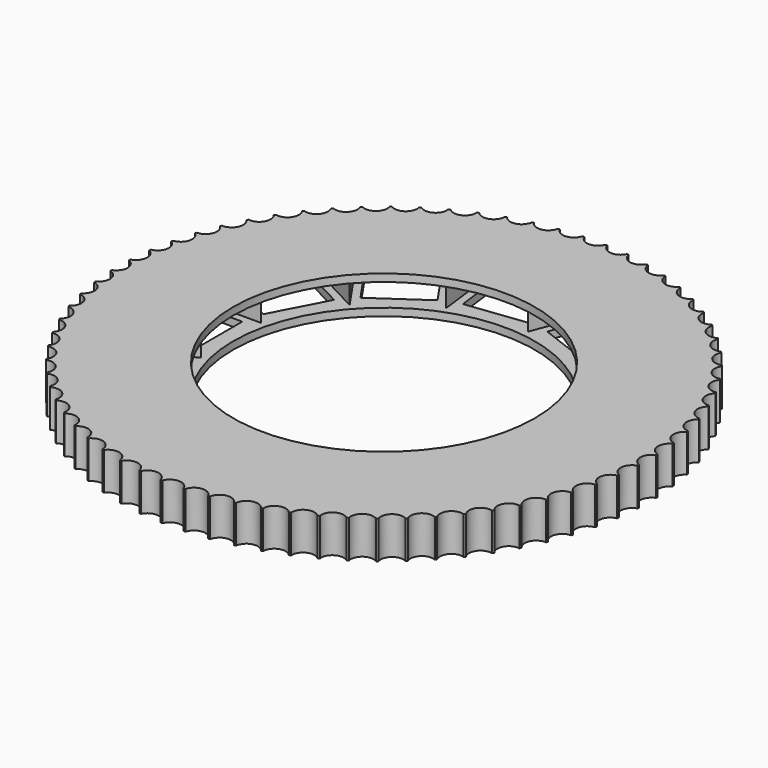
from build123d import *

# Parameters (mm, degrees)
F1_R          = 35
F1_R_2        = 20
F2_DEPTH      = 4
F2_DEPTH_BACK = 1
F0_W          = 10
F0_H          = 8
F3_DEPTH      = 3
F3_DEPTH_BACK = 1
F4_DEPTH      = 3
F5_R          = 1.5
F6_DEPTH      = 4.001
F6_DEPTH_BACK = 1.001


# Not quite as in the source:
# - a feature of the source that left no trace in its solid (it failed there, or was rolled back) is left out


with BuildPart() as f2:
    # F1 (on Top) → F2 (new body, two sides)
    with BuildSketch(Plane.XY) as f2_sk:
        Circle(F1_R)
        Circle(F1_R_2, mode=Mode.SUBTRACT)
    extrude(amount=F2_DEPTH)
    extrude(f2_sk.sketch, amount=-F2_DEPTH_BACK)

    # F0 (on Top) → F3 (cut, two sides)
    with BuildSketch(Plane.XY) as f3_sk:
        with Locations((-27, 0)):
            Rectangle(F0_W, F0_H)
        Polygon((-21.3389252525, -6.6820856824), (-30.1934855091, -11.3293174028), (-26.4757001327, -18.412965608), (-17.6211398762, -13.7657338876), align=None)
        Polygon((-15.7893598917, -15.8333860627), (-21.470007359, -24.0632247217), (-14.8861364318, -28.6077426955), (-9.2054889645, -20.3779040366), align=None)
        Polygon((-6.622642462, -21.3574485091), (-7.8280092646, -31.2845372501), (0.1136617282, -32.2488306922), (1.3190285308, -22.3217419512), align=None)
        Polygon((4.0612425442, -21.9887768872), (7.6072914146, -31.3389393141), (15.0874213561, -28.5021002178), (11.5413724857, -19.1519377909), align=None)
        Polygon((13.8147458268, -17.582741474), (21.2998533085, -24.2139680564), (26.6048345744, -18.225882071), (19.1197270927, -11.5946554886), align=None)
        Polygon((20.4034573262, -9.148711884), (30.1128755005, -11.5418685269), (32.0274008148, -3.7743339875), (22.3179826405, -1.3811773446), align=None)
        Polygon((22.3179826405, 1.3811773446), (32.0274008148, 3.7743339875), (30.1128755005, 11.5418685269), (20.4034573262, 9.148711884), align=None)
        Polygon((19.1197270927, 11.5946554886), (26.6048345744, 18.225882071), (21.2998533085, 24.2139680564), (13.8147458268, 17.582741474), align=None)
        Polygon((11.5413724857, 19.1519377909), (15.0874213561, 28.5021002178), (7.6072914146, 31.3389393141), (4.0612425442, 21.9887768872), align=None)
        Polygon((1.3190285308, 22.3217419512), (0.1136617282, 32.2488306922), (-7.8280092646, 31.2845372501), (-6.622642462, 21.3574485091), align=None)
        Polygon((-9.2054889645, 20.3779040366), (-14.8861364318, 28.6077426955), (-21.470007359, 24.0632247217), (-15.7893598917, 15.8333860627), align=None)
        Polygon((-17.6211398762, 13.7657338876), (-26.4757001327, 18.412965608), (-30.1934855091, 11.3293174028), (-21.3389252525, 6.6820856824), align=None)
    extrude(amount=F3_DEPTH, mode=Mode.SUBTRACT)
    extrude(f3_sk.sketch, amount=-F3_DEPTH_BACK, mode=Mode.SUBTRACT)

    # F0 (on Top) → F4 (cut)
    with BuildSketch(Plane.XY):
        Polygon((-20.2857974282, 5), (-33, 5), (-33, -5), (-20.2857974282, -5), (-10.7590933717, 0), align=None)
        with Locations((-27, 0)):
            Rectangle(F0_W, F0_H, mode=Mode.SUBTRACT)
        Polygon((-31.5436647068, 10.9085845492), (-20.2857974282, 5), (-9.5267040565, 5), (-15.6385657078, 13.8545602565), (-26.8964329863, 19.7631448057), align=None)
        Polygon((-30.1934855091, 11.3293174028), (-26.4757001327, 18.412965608), (-17.6211398762, 13.7657338876), (-21.3389252525, 6.6820856824), align=None, mode=Mode.SUBTRACT)
        Polygon((-9.5267040565, 5), (-20.2857974282, 5), (-10.7590933717, 0), (-7.3209820639, 1.8044600144), align=None)
        Polygon((-15.6385657078, 13.8545602565), (-9.5267040565, 5), (-5.6438333004, 5), (-6.1118616512, 8.8545602565), align=None)
        Polygon((-7.3209820639, -1.8044600144), (-10.7590933717, 0), (-20.2857974282, -5), (-9.5267040565, -5), align=None)
        Polygon((-9.5267040565, -5), (-20.2857974282, -5), (-31.5436647068, -10.9085845492), (-26.8964329863, -19.7631448057), (-15.6385657078, -13.8545602565), align=None)
        Polygon((-26.4757001327, -18.412965608), (-30.1934855091, -11.3293174028), (-21.3389252525, -6.6820856824), (-17.6211398762, -13.7657338876), align=None, mode=Mode.SUBTRACT)
        Polygon((-22.8610559716, 24.3181438408), (-15.6385657078, 13.8545602565), (-6.1118616512, 8.8545602565), (-7.4087270488, 19.5352077238), (-14.6312173127, 29.9987913081), align=None)
        Polygon((-21.470007359, 24.0632247217), (-14.8861364318, 28.6077426955), (-9.2054889645, 20.3779040366), (-15.7893598917, 15.8333860627), align=None, mode=Mode.SUBTRACT)
        Polygon((-5.6438333004, -5), (-9.5267040565, -5), (-15.6385657078, -13.8545602565), (-6.1118616512, -8.8545602565), align=None)
        Polygon((-7.4087270488, 19.5352077238), (-6.1118616512, 8.8545602565), (-2.6737503434, 7.0501002421), (-1.2968653976, 10.6806474673), align=None)
        Polygon((-6.1118616512, -8.8545602565), (-15.6385657078, -13.8545602565), (-22.8610559716, -24.3181438408), (-14.6312173127, -29.9987913081), (-7.4087270488, -19.5352077238), align=None)
        Polygon((-14.8861364318, -28.6077426955), (-21.470007359, -24.0632247217), (-15.7893598917, -15.8333860627), (-9.2054889645, -20.3779040366), align=None, mode=Mode.SUBTRACT)
        Polygon((-8.9412548189, 32.156709444), (-7.4087270488, 19.5352077238), (-1.2968653976, 10.6806474673), (2.5183616922, 20.7405745264), (0.9858339221, 33.3620762465), align=None)
        Polygon((-7.8280092646, 31.2845372501), (0.1136617282, 32.2488306922), (1.3190285308, 22.3217419512), (-6.622642462, 21.3574485091), align=None, mode=Mode.SUBTRACT)
        Polygon((-2.6737503434, -7.0501002421), (-6.1118616512, -8.8545602565), (-7.4087270488, -19.5352077238), (-1.2968653976, -10.6806474673), align=None)
        Polygon((2.5183616922, 20.7405745264), (-1.2968653976, 10.6806474673), (0.9088565951, 7.4851074817), (3.8152270897, 10.0599270591), align=None)
        Polygon((-1.2968653976, -10.6806474673), (-7.4087270488, -19.5352077238), (-8.9412548189, -32.156709444), (0.9858339221, -33.3620762465), (2.5183616922, -20.7405745264), align=None)
        Polygon((0.1136617282, -32.2488306922), (-7.8280092646, -31.2845372501), (-6.622642462, -21.3574485091), (1.3190285308, -22.3217419512), align=None, mode=Mode.SUBTRACT)
        Polygon((7.026880059, 32.6285604438), (2.5183616922, 20.7405745264), (3.8152270897, 10.0599270591), (11.868524119, 17.194525656), (16.3770424858, 29.0825115734), align=None)
        Polygon((7.6072914146, 31.3389393141), (15.0874213561, 28.5021002178), (11.5413724857, 19.1519377909), (4.0612425442, 21.9887768872), align=None, mode=Mode.SUBTRACT)
        Polygon((0.9088565951, -7.4851074817), (-1.2968653976, -10.6806474673), (2.5183616922, -20.7405745264), (3.8152270897, -10.0599270591), align=None)
        Polygon((11.868524119, 17.194525656), (3.8152270897, 10.0599270591), (4.2832554405, 6.2053668026), (8.0532970293, 7.1345985969), align=None)
        Polygon((3.8152270897, -10.0599270591), (2.5183616922, -20.7405745264), (7.026880059, -32.6285604438), (16.3770424858, -29.0825115734), (11.868524119, -17.194525656), align=None)
        Polygon((15.0874213561, -28.5021002178), (7.6072914146, -31.3389393141), (4.0612425442, -21.9887768872), (11.5413724857, -19.1519377909), align=None, mode=Mode.SUBTRACT)
        Polygon((21.3852413984, 25.6256014628), (11.868524119, 17.194525656), (8.0532970293, 7.1345985969), (18.4997507014, 9.7094181743), (28.0164679809, 18.1404939811), align=None)
        Polygon((21.2998533085, 24.2139680564), (26.6048345744, 18.225882071), (19.1197270927, 11.5946554886), (13.8147458268, 17.582741474), align=None, mode=Mode.SUBTRACT)
        Polygon((4.2832554405, -6.2053668026), (3.8152270897, -10.0599270591), (11.868524119, -17.194525656), (8.0532970293, -7.1345985969), align=None)
        Polygon((18.4997507014, 9.7094181743), (8.0532970293, 7.1345985969), (6.6764120834, 3.5040513717), (10.4464536722, 2.5748195774), align=None)
        Polygon((8.0532970293, -7.1345985969), (11.868524119, -17.194525656), (21.3852413984, -25.6256014628), (28.0164679809, -18.1404939811), (18.4997507014, -9.7094181743), align=None)
        Polygon((26.6048345744, -18.225882071), (21.2998533085, -24.2139680564), (13.8147458268, -17.582741474), (19.1197270927, -11.5946554886), align=None, mode=Mode.SUBTRACT)
        Polygon((30.8445016536, 12.7521260086), (18.4997507014, 9.7094181743), (10.4464536722, 2.5748195774), (20.8929073443, 0), (33.2376582965, 3.0427078344), align=None)
        Polygon((30.1128755005, 11.5418685269), (32.0274008148, 3.7743339875), (22.3179826405, 1.3811773446), (20.4034573262, 9.148711884), align=None, mode=Mode.SUBTRACT)
        Polygon((6.6764120834, -3.5040513717), (8.0532970293, -7.1345985969), (18.4997507014, -9.7094181743), (10.4464536722, -2.5748195774), align=None)
        Polygon((20.8929073443, 0), (10.4464536722, 2.5748195774), (7.5400831775, 0), (10.4464536722, -2.5748195774), align=None)
        Polygon((10.4464536722, -2.5748195774), (18.4997507014, -9.7094181743), (30.8445016536, -12.7521260086), (33.2376582965, -3.0427078344), (20.8929073443, 0), align=None)
        Polygon((32.0274008148, -3.7743339875), (30.1128755005, -11.5418685269), (20.4034573262, -9.148711884), (22.3179826405, -1.3811773446), align=None, mode=Mode.SUBTRACT)
    extrude(amount=F4_DEPTH, mode=Mode.SUBTRACT)

    # F5 (on Top) → F6 (cut, two sides)
    with BuildSketch(Plane.XY) as f6_sk:
        with Locations((-35.5, 0)):
            Circle(F5_R)
        with Locations((-35.3649117823, -3.0940288675)):
            Circle(F5_R)
        with Locations((-34.9606752319, -6.1645103072)):
            Circle(F5_R)
        with Locations((-34.2903668333, -9.1880761011)):
            Circle(F5_R)
        with Locations((-33.3590880379, -12.1417150881)):
            Circle(F5_R)
        with Locations((-32.1739264398, -15.0029482918)):
            Circle(F5_R)
        with Locations((-30.7439018343, -17.75)):
            Circle(F5_R)
        with Locations((-29.0798975723, -20.3619634905)):
            Circle(F5_R)
        with Locations((-27.1945777307, -22.8189601439)):
            Circle(F5_R)
        with Locations((-25.1022907321, -25.1022907321)):
            Circle(F5_R)
        with Locations((-22.8189601439, -27.1945777307)):
            Circle(F5_R)
        with Locations((-20.3619634905, -29.0798975723)):
            Circle(F5_R)
        with Locations((-17.75, -30.7439018343)):
            Circle(F5_R)
        with Locations((-15.0029482918, -32.1739264398)):
            Circle(F5_R)
        with Locations((-12.1417150881, -33.3590880379)):
            Circle(F5_R)
        with Locations((-9.1880761011, -34.2903668333)):
            Circle(F5_R)
        with Locations((-6.1645103072, -34.9606752319)):
            Circle(F5_R)
        with Locations((-3.0940288675, -35.3649117823)):
            Circle(F5_R)
        with Locations((0, -35.5)):
            Circle(F5_R)
        with Locations((3.0940288675, -35.3649117823)):
            Circle(F5_R)
        with Locations((6.1645103072, -34.9606752319)):
            Circle(F5_R)
        with Locations((9.1880761011, -34.2903668333)):
            Circle(F5_R)
        with Locations((12.1417150881, -33.3590880379)):
            Circle(F5_R)
        with Locations((15.0029482918, -32.1739264398)):
            Circle(F5_R)
        with Locations((17.75, -30.7439018343)):
            Circle(F5_R)
        with Locations((20.3619634905, -29.0798975723)):
            Circle(F5_R)
        with Locations((22.8189601439, -27.1945777307)):
            Circle(F5_R)
        with Locations((25.1022907321, -25.1022907321)):
            Circle(F5_R)
        with Locations((27.1945777307, -22.8189601439)):
            Circle(F5_R)
        with Locations((29.0798975723, -20.3619634905)):
            Circle(F5_R)
        with Locations((30.7439018343, -17.75)):
            Circle(F5_R)
        with Locations((32.1739264398, -15.0029482918)):
            Circle(F5_R)
        with Locations((33.3590880379, -12.1417150881)):
            Circle(F5_R)
        with Locations((34.2903668333, -9.1880761011)):
            Circle(F5_R)
        with Locations((34.9606752319, -6.1645103072)):
            Circle(F5_R)
        with Locations((35.3649117823, -3.0940288675)):
            Circle(F5_R)
        with Locations((35.5, 0)):
            Circle(F5_R)
        with Locations((35.3649117823, 3.0940288675)):
            Circle(F5_R)
        with Locations((34.9606752319, 6.1645103072)):
            Circle(F5_R)
        with Locations((34.2903668333, 9.1880761011)):
            Circle(F5_R)
        with Locations((33.3590880379, 12.1417150881)):
            Circle(F5_R)
        with Locations((32.1739264398, 15.0029482918)):
            Circle(F5_R)
        with Locations((30.7439018343, 17.75)):
            Circle(F5_R)
        with Locations((29.0798975723, 20.3619634905)):
            Circle(F5_R)
        with Locations((27.1945777307, 22.8189601439)):
            Circle(F5_R)
        with Locations((25.1022907321, 25.1022907321)):
            Circle(F5_R)
        with Locations((22.8189601439, 27.1945777307)):
            Circle(F5_R)
        with Locations((20.3619634905, 29.0798975723)):
            Circle(F5_R)
        with Locations((17.75, 30.7439018343)):
            Circle(F5_R)
        with Locations((15.0029482918, 32.1739264398)):
            Circle(F5_R)
        with Locations((12.1417150881, 33.3590880379)):
            Circle(F5_R)
        with Locations((9.1880761011, 34.2903668333)):
            Circle(F5_R)
        with Locations((6.1645103072, 34.9606752319)):
            Circle(F5_R)
        with Locations((3.0940288675, 35.3649117823)):
            Circle(F5_R)
        with Locations((0, 35.5)):
            Circle(F5_R)
        with Locations((-3.0940288675, 35.3649117823)):
            Circle(F5_R)
        with Locations((-6.1645103072, 34.9606752319)):
            Circle(F5_R)
        with Locations((-9.1880761011, 34.2903668333)):
            Circle(F5_R)
        with Locations((-12.1417150881, 33.3590880379)):
            Circle(F5_R)
        with Locations((-15.0029482918, 32.1739264398)):
            Circle(F5_R)
        with Locations((-17.75, 30.7439018343)):
            Circle(F5_R)
        with Locations((-20.3619634905, 29.0798975723)):
            Circle(F5_R)
        with Locations((-22.8189601439, 27.1945777307)):
            Circle(F5_R)
        with Locations((-25.1022907321, 25.1022907321)):
            Circle(F5_R)
        with Locations((-27.1945777307, 22.8189601439)):
            Circle(F5_R)
        with Locations((-29.0798975723, 20.3619634905)):
            Circle(F5_R)
        with Locations((-30.7439018343, 17.75)):
            Circle(F5_R)
        with Locations((-32.1739264398, 15.0029482918)):
            Circle(F5_R)
        with Locations((-33.3590880379, 12.1417150881)):
            Circle(F5_R)
        with Locations((-34.2903668333, 9.1880761011)):
            Circle(F5_R)
        with Locations((-34.9606752319, 6.1645103072)):
            Circle(F5_R)
        with Locations((-35.3649117823, 3.0940288675)):
            Circle(F5_R)
    extrude(amount=F6_DEPTH, mode=Mode.SUBTRACT)
    extrude(f6_sk.sketch, amount=-F6_DEPTH_BACK, mode=Mode.SUBTRACT)


solid = f2.part
